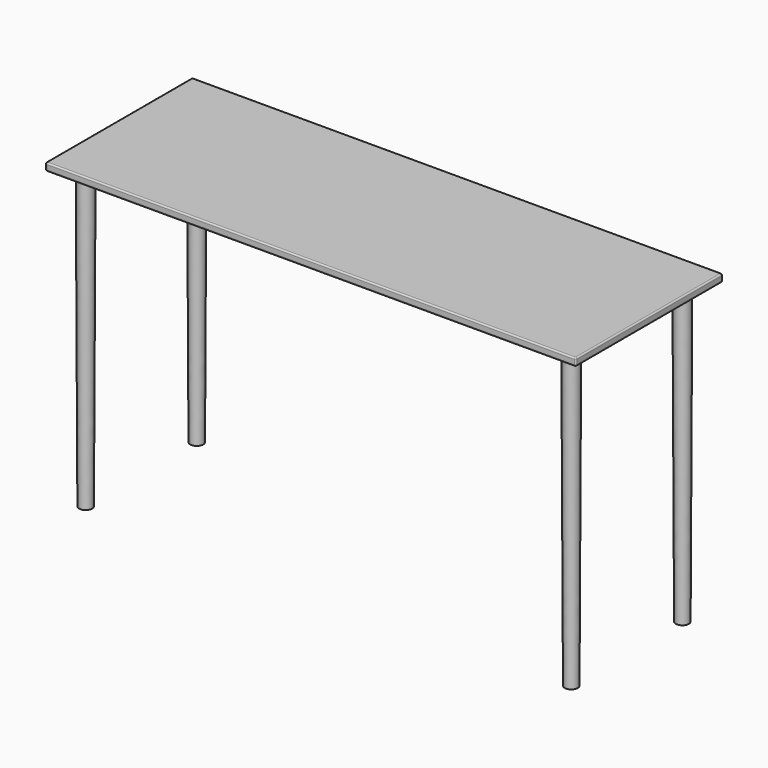
from build123d import *

# Parameters (mm, degrees)
F0_W     = 1879.6
F0_H     = 650.875
F1_DEPTH = 26.9875
F2_R     = 5.08
F3_R     = 27.559
F4_DEPTH = 1052.5125
F4_TAPER = 0.25
F5_SCALE = 0.05


with BuildPart() as f1:
    # F0 (on Top) → F1 (new body)
    with BuildSketch(Plane.XY):
        Rectangle(F0_W, F0_H)
    extrude(amount=F1_DEPTH)

    # F2
    f2_edges = [f1.edges().sort_by_distance(p)[0] for p in [
        (-939.8, 325.4375, 13.49375),
        (-939.8, -325.4375, 13.49375),
        (939.8, -325.4375, 13.49375),
        (0, -325.4375, 0),
        (0, -325.4375, 26.9875),
        (-939.8, 0, 0),
        (-939.8, 0, 26.9875),
        (939.8, 325.4375, 13.49375),
        (0, 325.4375, 0),
        (0, 325.4375, 26.9875),
        (939.8, 0, 0),
        (939.8, 0, 26.9875),
    ]]
    fillet(f2_edges, radius=F2_R)

    # F3 (on face) → F4 (join)
    with BuildSketch(Plane(origin=(0, 0, 0), x_dir=(1, 0, 0), z_dir=(0, 0, -1))):
        with Locations((-860.425, 246.0625)):
            Circle(F3_R)
        with Locations((-860.425, -246.0625)):
            Circle(F3_R)
        with Locations((860.425, 246.0625)):
            Circle(F3_R)
        with Locations((860.425, -246.0625)):
            Circle(F3_R)
    extrude(amount=F4_DEPTH, taper=F4_TAPER)


with BuildPart() as f1_1:
    # F5: moved
    add(f1.part.scale(F5_SCALE))


solid = f1_1.part
